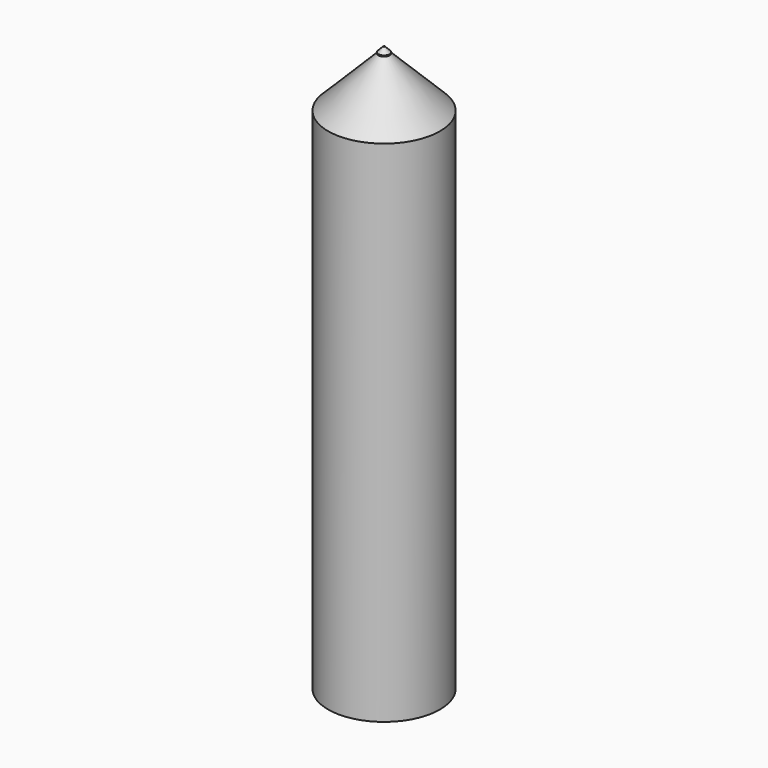
from build123d import *

# Parameters (mm, degrees)
F0_R     = 25.4
F1_DEPTH = 127
F2_SIZE  = 22.86
F4_DEPTH = 254.001
F5_R     = 2.54
F5_R_2   = 0.3020400554
F6_DEPTH = 129.794


# Not quite as in the source:
# - a fillet or chamfer that OpenCascade refuses, or shapes differently, is made with other operations: its cross-section is extruded or revolved along the edge and cut away or added


with BuildPart() as f1:
    # F0 (on Top) → F1 (new body, symmetric)
    with BuildSketch(Plane.XY):
        Circle(F0_R)
    extrude(amount=F1_DEPTH, both=True)

    # F2
    f2_edges = [f1.edges().sort_by_distance(p)[0] for p in [
        (-25.4, 0, 127),
    ]]
    chamfer(f2_edges, length=F2_SIZE)

    # F4 (cut, through all): a face of the model
    f4_faces = [f1.faces().sort_by_distance(p)[0] for p in [
        (0, 0, 127),
    ]]
    extrude(f4_faces, amount=-F4_DEPTH, mode=Mode.SUBTRACT)

    # F5 (on Top) → F6 (join, symmetric)
    with BuildSketch(Plane.XY):
        Circle(F5_R)
        Circle(F5_R_2, mode=Mode.SUBTRACT)
    extrude(amount=F6_DEPTH, both=True)

    # F7: chamfer of 2.286 on 1 edges, made by hand

    # F7_s1 → F7_t2 (revolve, cut)
    with BuildSketch(Plane.XZ):
        Polygon((0.254, 129.794), (2.54, 127.508), (2.54, 129.794), align=None)
    revolve(axis=Axis((0, 0, 129.794), (0, 0, 1)), mode=Mode.SUBTRACT)


solid = f1.part
